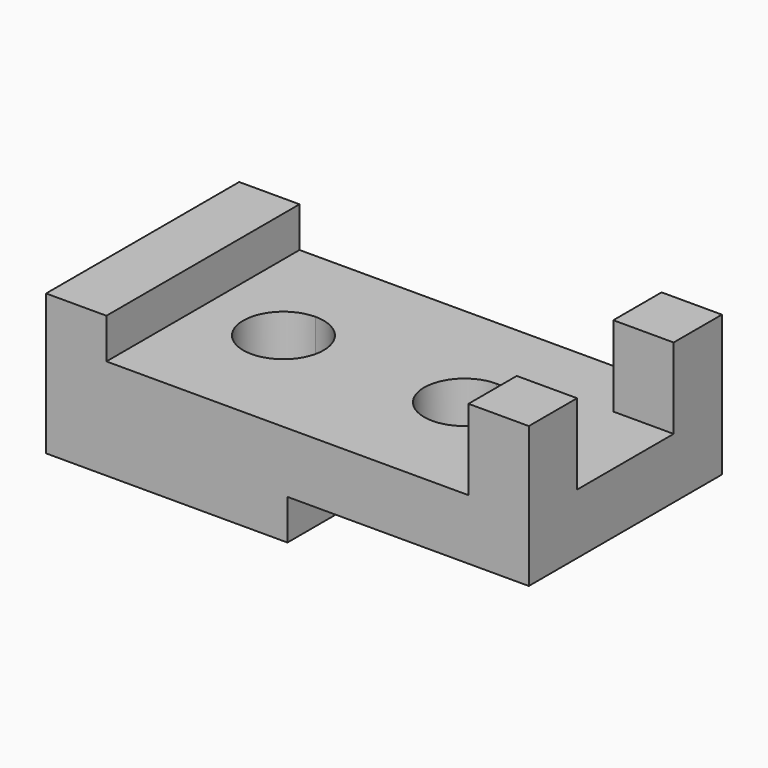
from build123d import *

# Parameters (mm, degrees)
F0_W     = 120
F0_H     = 60
F1_DEPTH = 25
F2_W     = 60
F2_H     = 60
F3_DEPTH = 10
F4_W     = 15
F4_H     = 60
F5_DEPTH = 10
F6_W     = 15
F6_H     = 15
F7_DEPTH = 20
F9_DEPTH = 25.001


with BuildPart() as f1:
    # F0 (on Top) → F1 (new body)
    with BuildSketch(Plane.XY):
        Rectangle(F0_W, F0_H)
    extrude(amount=F1_DEPTH)

    # F2 (on face) → F3 (cut)
    with BuildSketch(Plane(origin=(0, 0, 0), x_dir=(1, 0, 0), z_dir=(0, 0, -1))):
        with Locations((30, 0)):
            Rectangle(F2_W, F2_H)
    extrude(amount=-F3_DEPTH, mode=Mode.SUBTRACT)

    # F4 (on face) → F5 (join)
    with BuildSketch(Plane.XY.offset(25)):
        with Locations((-52.5, 0)):
            Rectangle(F4_W, F4_H)
    extrude(amount=F5_DEPTH)

    # F6 (on face) → F7 (join)
    with BuildSketch(Plane.XY.offset(25)):
        with Locations((52.5, -22.5)):
            Rectangle(F6_W, F6_H)
        with Locations((52.5, 22.5)):
            Rectangle(F6_W, F6_H)
    extrude(amount=F7_DEPTH)

    # F8 (on face) → F9 (cut, through all)
    with BuildSketch(Plane.XY.offset(25)):
        with BuildLine():
            Line((-25, 10), (-25, -10))
            ThreePointArc((-25, -10), (-17.9289321881, -7.0710678119), (-15, 0))
            ThreePointArc((-15, 0), (-17.9289321881, 7.0710678119), (-25, 10))
        make_face()
        with BuildLine():
            ThreePointArc((-25, 10), (-35, 0), (-25, -10))
            Line((-25, -10), (-25, 10))
        make_face()
        with BuildLine():
            ThreePointArc((20, 10), (10, 0), (20, -10))
            Line((20, -10), (20, 10))
        make_face()
        with BuildLine():
            Line((20, 10), (20, -10))
            ThreePointArc((20, -10), (27.0710678119, -7.0710678119), (30, 0))
            ThreePointArc((30, 0), (27.0710678119, 7.0710678119), (20, 10))
        make_face()
    extrude(amount=-F9_DEPTH, mode=Mode.SUBTRACT)


solid = f1.part
